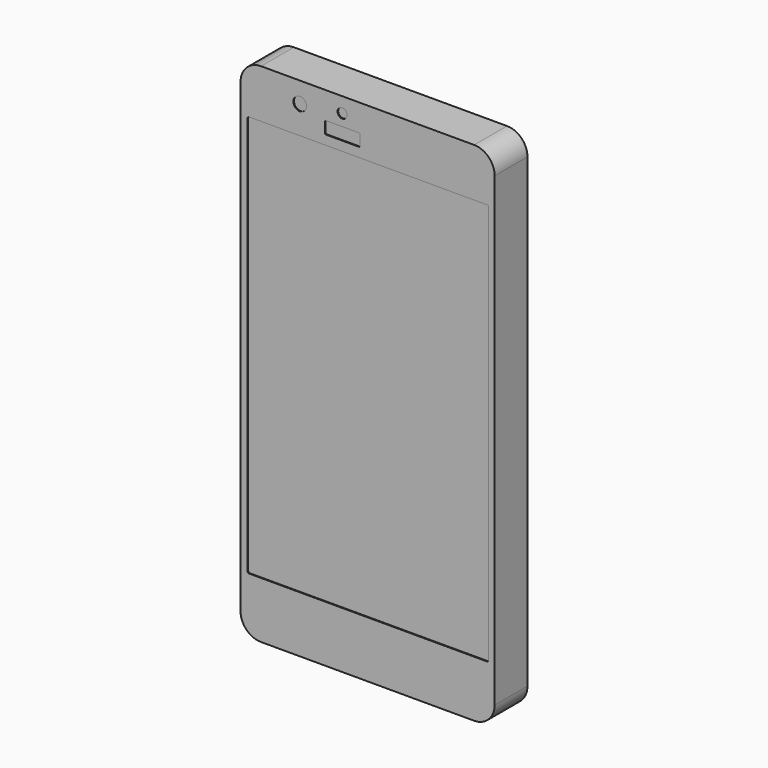
from build123d import *

# Parameters (mm, degrees)
F1_DEPTH = 12.7
F2_R     = 2.048268854
F2_R_2   = 1.4747920456
F3_DEPTH = 0.254


# Not quite as in the source:
# - a feature names something its author has since deleted; it is built from what else it names
# - the program builds the solid bodies; features that only make, move or delete a surface that nothing else refers to are left out


with BuildPart() as f1:
    # F0 (on Front) → F1 (new body)
    with BuildSketch(Plane.XZ):
        with BuildLine():
            Line((40.8309073806, 93.5981370211), (-25.1690926194, 93.5981370211))
            ThreePointArc((-25.1690926194, 93.5981370211), (-29.65922068, 91.7382650816), (-31.5190926194, 87.2481370211))
            Line((-31.5190926194, 87.2481370211), (-31.5190926194, -57.0518629789))
            ThreePointArc((-31.5190926194, -57.0518629789), (-29.65922068, -61.5419910395), (-25.1690926194, -63.4018629789))
            Line((-25.1690926194, -63.4018629789), (40.8309073806, -63.4018629789))
            ThreePointArc((40.8309073806, -63.4018629789), (45.3210354411, -61.5419910395), (47.1809073806, -57.0518629789))
            Line((47.1809073806, -57.0518629789), (47.1809073806, 87.2481370211))
            ThreePointArc((47.1809073806, 87.2481370211), (45.3210354411, 91.7382650816), (40.8309073806, 93.5981370211))
        make_face()
    extrude(amount=F1_DEPTH)

    # F2 (on face) → F3 (cut)
    with BuildSketch(Plane.XZ.offset(12.7)):
        with Locations((-13.1258289722, 87.2481370211)):
            Circle(F2_R)
        with Locations((0, 88.9561623335)):
            Circle(F2_R_2)
        with BuildLine():
            Line((5.0678964471, 85.2992907166), (-4.9437066773, 85.2992907166))
            ThreePointArc((-4.9437066773, 85.2992907166), (-5.2614981956, 85.1676571598), (-5.3931317525, 84.8498656414))
            Line((-5.3931317525, 84.8498656414), (-5.3931317525, 81.9237329997))
            ThreePointArc((-5.3931317525, 81.9237329997), (-5.2614981956, 81.6059414814), (-4.9437066773, 81.4743079245))
            Line((-4.9437066773, 81.4743079245), (5.0678964471, 81.4743079245))
            ThreePointArc((5.0678964471, 81.4743079245), (5.3856879655, 81.6059414814), (5.5173215223, 81.9237329997))
            Line((5.5173215223, 81.9237329997), (5.5173215223, 84.8498656414))
            ThreePointArc((5.5173215223, 84.8498656414), (5.3856879655, 85.1676571598), (5.0678964471, 85.2992907166))
        make_face()
        with BuildLine():
            Line((44.9024620466, 78.5618498921), (-28.8875750266, 78.5618498921))
            ThreePointArc((-28.8875750266, 78.5618498921), (-29.2053665449, 78.4302163352), (-29.3370001018, 78.1124248169))
            Line((-29.3370001018, 78.1124248169), (-29.3370001018, -45.495712664))
            ThreePointArc((-29.3370001018, -45.495712664), (-29.2053665449, -45.8135041823), (-28.8875750266, -45.9451377392))
            Line((-28.8875750266, -45.9451377392), (44.9024620466, -45.9451377392))
            ThreePointArc((44.9024620466, -45.9451377392), (45.2202535649, -45.8135041823), (45.3518871218, -45.495712664))
            Line((45.3518871218, -45.495712664), (45.3518871218, 78.1124248169))
            ThreePointArc((45.3518871218, 78.1124248169), (45.2202535649, 78.4302163352), (44.9024620466, 78.5618498921))
        make_face()
    extrude(amount=-F3_DEPTH, mode=Mode.SUBTRACT)


solid = f1.part
